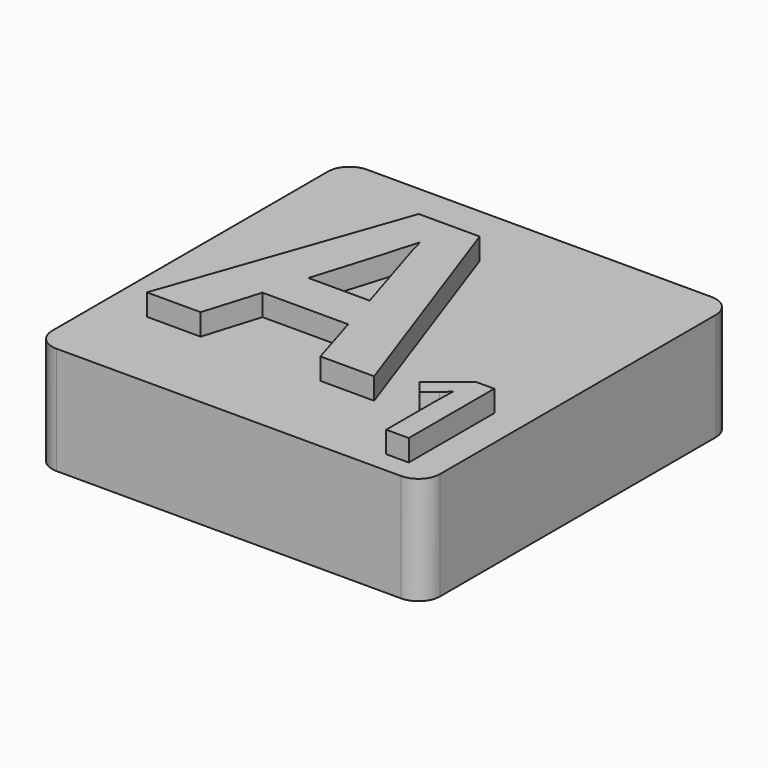
from build123d import *

# Parameters (mm, degrees)
F0_W           = 18
F0_H           = 18
F1_DEPTH       = 5
F2_W           = 16
F2_H           = 16
F3_DEPTH       = 3
F4_TEXT_SIZE   = 15.2777777778
F4_TEXT_SIZE_2 = 6.9444444444
F5_DEPTH       = 1
F6_R           = 1


# Not quite as in the source:
# - Text() gives the source's letters only with a copy of the font that has no kerning and outlines rounded to 1/6400 em; it was checked with that copy


with BuildPart() as f1:
    # F0 (on Top) → F1 (new body)
    with BuildSketch(Plane.XY):
        with Locations((5.0695089158, -1.7574313941)):
            Rectangle(F0_W, F0_H)
    extrude(amount=F1_DEPTH)

    # F2 (on Top) → F3 (cut)
    with BuildSketch(Plane.XY):
        with Locations((5.0695089158, -1.7574313941)):
            Rectangle(F2_W, F2_H)
    extrude(amount=F3_DEPTH, mode=Mode.SUBTRACT)

    # F4 (on face) → F5 (join)
    with BuildSketch(Plane.XY.offset(5)):
        with Locations((-1.9304910842, -6.7574313941)):
            Text('A', F4_TEXT_SIZE, font='Open Sans', font_style=FontStyle.BOLD, text_align=(TextAlign.LEFT, TextAlign.BOTTOM))
        with Locations((9.7502814852, -9.7574313941)):
            Text('1', F4_TEXT_SIZE_2, font='Open Sans', font_style=FontStyle.BOLD, text_align=(TextAlign.LEFT, TextAlign.BOTTOM))
    extrude(amount=F5_DEPTH)

    # F6
    f6_edges = [f1.edges().sort_by_distance(p)[0] for p in [
        (14.069509, 7.242569, 2.5),
        (14.069509, -10.757431, 2.5),
        (-3.930491, -10.757431, 2.5),
        (-3.930491, 7.242569, 2.5),
        (13.069509, -9.757431, 1.5),
        (-2.930491, -9.757431, 1.5),
        (-2.930491, 6.242569, 1.5),
        (13.069509, 6.242569, 1.5),
    ]]
    fillet(f6_edges, radius=F6_R)


solid = f1.part
